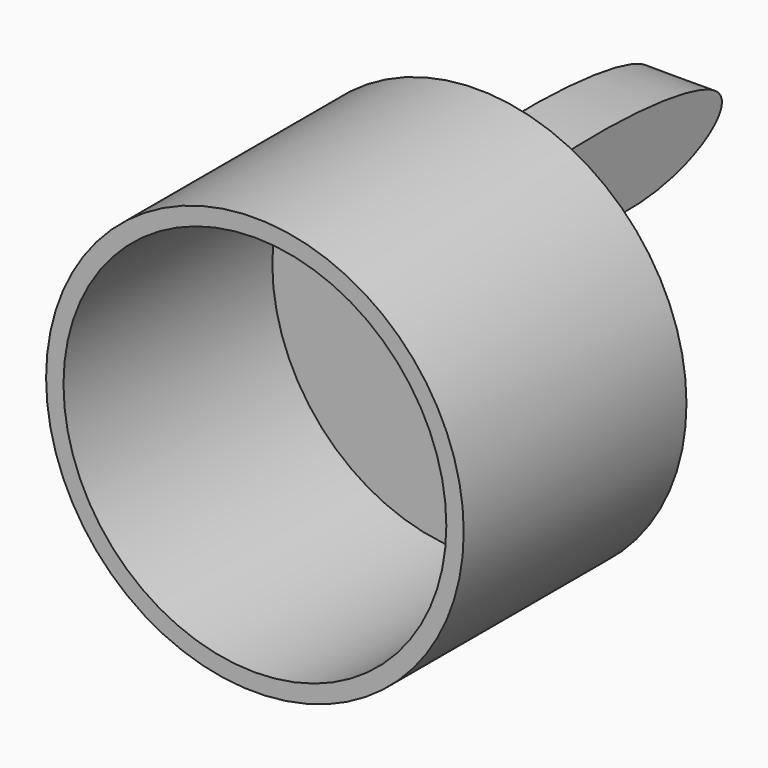
from build123d import *

# Parameters (mm, degrees)
F0_R     = 76.2
F0_R_2   = 69.85
F1_DEPTH = 25.4
F2_DEPTH = 76.2
F3_R     = 70.0511515775
F4_DEPTH = 6.35
F6_DEPTH = 25.4


with BuildPart() as f1:
    # F0 (on Front) → F1 (new body)
    with BuildSketch(Plane.XZ):
        Circle(F0_R)
        Circle(F0_R_2, mode=Mode.SUBTRACT)
    extrude(amount=F1_DEPTH)

    # F2 (add): a face of the model
    f2_faces = [f1.faces().sort_by_distance(p)[0] for p in [
        (-74.0447385309, -25.4, 0),
    ]]
    extrude(f2_faces, amount=F2_DEPTH)

    # F3 (on Front) → F4 (join)
    with BuildSketch(Plane.XZ):
        Circle(F3_R)
    extrude(amount=F4_DEPTH)

    # F5 (on Right) → F6 (join)
    with BuildSketch(Plane.YZ):
        with BuildLine():
            add(Edge.make_bspline(
                [(-27.6209320873, 52.8044328094), (-19.1718805943, 63.260073286), (113.9909728332, 64.3613693038), (44.95583544, 16.606444594), (-34.7977200102, 43.9232093535), (-27.6209320873, 52.8044328094)],
                knots=[0, 0, 0, 0, 0.4070795235, 0.6542187711, 1, 1, 1, 1], degree=3))
        make_face()
    extrude(amount=F6_DEPTH)


solid = f1.part
